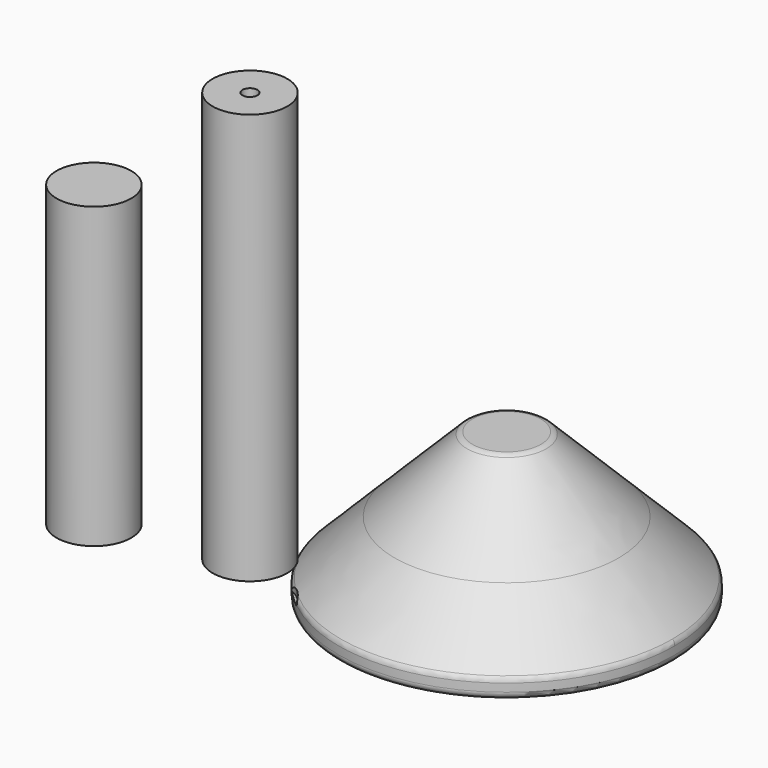
from build123d import *

# Parameters (mm, degrees)
F0_R          = 50
F1_DEPTH      = 600
F2_R          = 10
F3_DEPTH      = 20
F4_DEPTH      = 400
F0_W          = 100
F0_H          = 100
F5_DEPTH      = 30
F6_R          = 7.5
F7_DEPTH      = 200
F8_DEPTH      = 100
F9_R          = 225
F9_R_2        = 150
F10_DEPTH     = 50
F11_DEPTH     = 50
F12_SIZE      = 74.999
F9_W          = 100
F9_H          = 100
F13_DEPTH     = 50
F14_T3_DEPTH  = 155
F14_S4_R      = 7.5
F14_T5_DEPTH  = 87
F14_T8_DEPTH  = 155
F14_S9_R      = 7.5
F14_T10_DEPTH = 87
F14_T13_DEPTH = 155
F14_S14_R     = 7.5
F14_T15_DEPTH = 87
F14_T18_DEPTH = 155
F14_S19_R     = 7.5
F14_T20_DEPTH = 87
F15_DEPTH     = 50
F16_DEPTH     = 100
F17_SIZE      = 99.9999
F18_R         = 10


# Not quite as in the source:
# - a fillet or chamfer that OpenCascade refuses, or shapes differently, is made with other operations: its cross-section is extruded or revolved along the edge and cut away or added
# - a fillet or chamfer is up to 0.001 mm smaller than in the source, because OpenCascade refuses the exact size


with BuildPart() as f1:
    # F0 (on Top) → F1 (new body)
    with BuildSketch(Plane.XY):
        with Locations((-98.0170294642, -16.0204097629)):
            Circle(F0_R)
    extrude(amount=F1_DEPTH)

    # F2 (on face) → F3 (cut)
    with BuildSketch(Plane.XY.offset(600)):
        with Locations((-98.0170294642, -16.0204097629)):
            Circle(F2_R)
    extrude(amount=-F3_DEPTH, mode=Mode.SUBTRACT)


with BuildPart() as f4:
    # F0 (on Top) → F4 (new body)
    with BuildSketch(Plane.XY):
        with Locations((-335.2196514606, 19.3492192775)):
            Circle(F0_R)
    extrude(amount=F4_DEPTH)


with BuildPart() as f5:
    # F0 (on Top) → F5 (new body)
    with BuildSketch(Plane.XY):
        with Locations((87.0656251907, 182.166326046)):
            Rectangle(F0_W, F0_H)
    extrude(amount=F5_DEPTH)

    # F6 (on face) → F7 (join)
    with BuildSketch(Plane.YZ.offset(137.0656251907)):
        with Locations((182.166326046, 15)):
            Circle(F6_R)
    extrude(amount=-F7_DEPTH)

    # F6 (on face) → F8 (join)
    with BuildSketch(Plane.YZ.offset(137.0656251907)):
        with Locations((182.166326046, 15)):
            Circle(F6_R)
    extrude(amount=F8_DEPTH)

    # F9 (on face) → F10 (join)
    with BuildSketch(Plane.XY.offset(30)):
        with Locations((87.0656251907, 182.166326046)):
            Circle(F9_R)
        with Locations((87.0656251907, 182.166326046)):
            Circle(F9_R_2, mode=Mode.SUBTRACT)
    extrude(amount=-F10_DEPTH)

    # F11 (add): a face of the model
    f11_faces = [f5.faces().sort_by_distance(p)[0] for p in [
        (-131.5704137786, 182.166326046, 30),
    ]]
    extrude(f11_faces, amount=F11_DEPTH)

    # F12 (size 75 in the source; OpenCascade refuses exactly that, so slightly less here)
    f12_edges = [f5.edges().sort_by_distance(p)[0] for p in [
        (-137.934375, 182.166326, 30),
        (-137.934375, 182.166326, 80),
    ]]
    chamfer(f12_edges, length=F12_SIZE)

    # F9 (on face) → F13 (join)
    with BuildSketch(Plane.XY.offset(30)):
        with Locations((87.0656251907, 182.166326046)):
            Circle(F9_R_2)
        with Locations((87.0656251907, 182.166326046)):
            Rectangle(F9_W, F9_H, mode=Mode.SUBTRACT)
        with Locations((87.0656251907, 182.166326046)):
            Rectangle(F9_W, F9_H)
    extrude(amount=F13_DEPTH)

    # F14: fillet of radius 50 on 4 edges, made by hand


with BuildPart() as f14_tool1:
    # F14_s2 → F14_t3 (new body)
    with BuildSketch(Plane.XY.offset(-125)):
        with BuildLine():
            ThreePointArc((137.0656251907, 182.166326046), (122.4209642501, 146.8109869867), (87.0656251907, 132.166326046))
            Line((87.0656251907, 132.166326046), (137.0656251907, 132.166326046))
            Line((137.0656251907, 132.166326046), (137.0656251907, 182.166326046))
        make_face()
    extrude(amount=F14_T3_DEPTH)

    # F14_s4 → F14_t5 (cut, symmetric)
    with BuildSketch(Plane.YZ.offset(112.1)):
        with Locations((182.166326046, 15)):
            Circle(F14_S4_R)
    extrude(amount=F14_T5_DEPTH, both=True, mode=Mode.SUBTRACT)


with BuildPart() as f14_tool6:
    # F14_s7 → F14_t8 (new body)
    with BuildSketch(Plane.XY.offset(-125)):
        with BuildLine():
            ThreePointArc((137.0656251907, 182.166326046), (122.4209642501, 217.5216651053), (87.0656251907, 232.166326046))
            Line((87.0656251907, 232.166326046), (137.0656251907, 232.166326046))
            Line((137.0656251907, 232.166326046), (137.0656251907, 182.166326046))
        make_face()
    extrude(amount=F14_T8_DEPTH)

    # F14_s9 → F14_t10 (cut, symmetric)
    with BuildSketch(Plane.YZ.offset(112.1)):
        with Locations((182.166326046, 15)):
            Circle(F14_S9_R)
    extrude(amount=F14_T10_DEPTH, both=True, mode=Mode.SUBTRACT)


with BuildPart() as f14_tool11:
    # F14_s12 → F14_t13 (new body)
    with BuildSketch(Plane.XY.offset(-125)):
        with BuildLine():
            ThreePointArc((37.0656251907, 182.166326046), (51.7102861314, 146.8109869867), (87.0656251907, 132.166326046))
            Line((87.0656251907, 132.166326046), (37.0656251907, 132.166326046))
            Line((37.0656251907, 132.166326046), (37.0656251907, 182.166326046))
        make_face()
    extrude(amount=F14_T13_DEPTH)

    # F14_s14 → F14_t15 (cut, symmetric)
    with BuildSketch(Plane.YZ.offset(62.1)):
        with Locations((182.166326046, 15)):
            Circle(F14_S14_R)
    extrude(amount=F14_T15_DEPTH, both=True, mode=Mode.SUBTRACT)


with BuildPart() as f14_tool16:
    # F14_s17 → F14_t18 (new body)
    with BuildSketch(Plane.XY.offset(-125)):
        with BuildLine():
            ThreePointArc((87.0656251907, 232.166326046), (51.7102861314, 217.5216651053), (37.0656251907, 182.166326046))
            Line((37.0656251907, 182.166326046), (37.0656251907, 232.166326046))
            Line((37.0656251907, 232.166326046), (87.0656251907, 232.166326046))
        make_face()
    extrude(amount=F14_T18_DEPTH)

    # F14_s19 → F14_t20 (cut, symmetric)
    with BuildSketch(Plane.YZ.offset(62.1)):
        with Locations((182.166326046, 15)):
            Circle(F14_S19_R)
    extrude(amount=F14_T20_DEPTH, both=True, mode=Mode.SUBTRACT)


with BuildPart() as f5_1:
    add(f5.part)

    # F14_t21: cut F14_tool1, F14_tool6, F14_tool11, F14_tool16
    add([f14_tool1.part, f14_tool6.part, f14_tool11.part, f14_tool16.part], mode=Mode.SUBTRACT)


with BuildPart() as f15_tool:
    # F0 (on Top) → F15 (new body)
    with BuildSketch(Plane.XY):
        with Locations((-98.0170294642, -16.0204097629)):
            Circle(F0_R)
    extrude(amount=F15_DEPTH)


with BuildPart() as f1_1:
    add(f1.part)

    # F15: cut by f15_tool
    add(f15_tool.part, mode=Mode.SUBTRACT)


with BuildPart() as f5_2:
    add(f5_1.part)

    # F15: cut by f15_tool
    add(f15_tool.part, mode=Mode.SUBTRACT)

    # F16 (add): a face of the model
    f16_faces = [f5_2.faces().sort_by_distance(p)[0] for p in [
        (87.0656252182, 182.166326046, 80),
    ]]
    extrude(f16_faces, amount=F16_DEPTH)

    # F17 (size 100 in the source; OpenCascade refuses exactly that, so slightly less here)
    f17_edges = [f5_2.edges().sort_by_distance(p)[0] for p in [
        (-62.935375, 182.166326, 180),
    ]]
    chamfer(f17_edges, length=F17_SIZE)

    # F18
    f18_edges = [f5_2.edges().sort_by_distance(p)[0] for p in [
        (-137.934375, 182.166326, -20),
        (5.506534, 391.864, 5.001),
        (184.657734, -20.566947, 5.001),
        (37.064516, 182.166657, 180),
    ]]
    fillet(f18_edges, radius=F18_R)


solid = Compound([f4.part, f1_1.part, f5_2.part])
